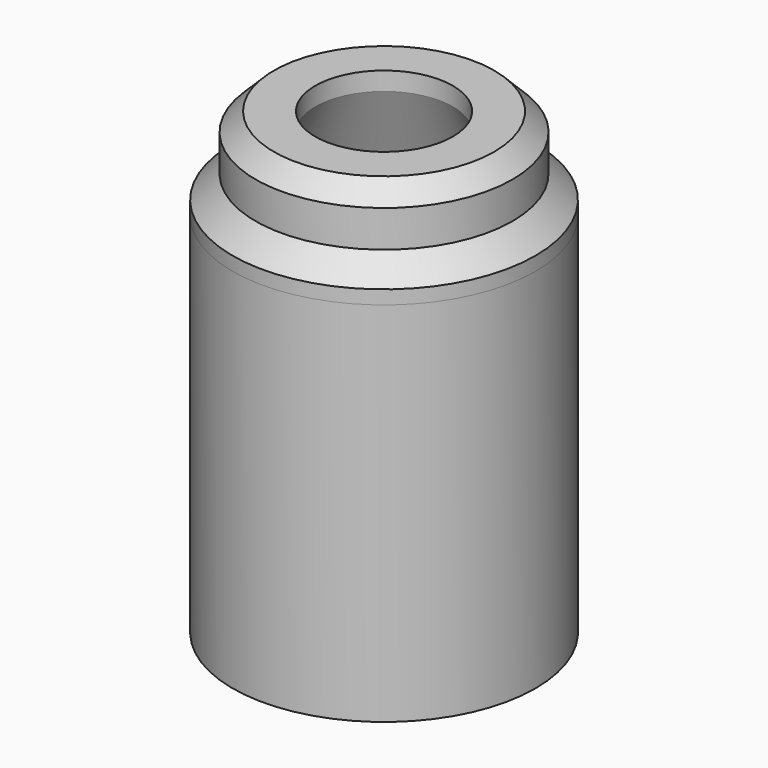
from build123d import *

# Parameters (mm, degrees)
F0_R          = 16.5
F0_R_2        = 14
F1_DEPTH      = 40
F2_R          = 14
F2_R_2        = 7.5
F3_DEPTH      = 10
F3_DEPTH_BACK = 5
F4_S5_R       = 16.5
F4_T6_DEPTH   = 27
F5_SIZE       = 2
F6_S5_R       = 14
F6_T6_DEPTH   = 24
F7_SIZE       = 5


# Not quite as in the source:
# - a fillet or chamfer that OpenCascade refuses, or shapes differently, is made with other operations: its cross-section is extruded or revolved along the edge and cut away or added


with BuildPart() as f1:
    # F0 (on Top) → F1 (new body)
    with BuildSketch(Plane.XY):
        Circle(F0_R)
        Circle(F0_R_2, mode=Mode.SUBTRACT)
    extrude(amount=F1_DEPTH)

    # F2 (on face) → F3 (join, two sides)
    with BuildSketch(Plane.XY.offset(40)) as f3_sk:
        Circle(F2_R)
        Circle(F2_R_2, mode=Mode.SUBTRACT)
    extrude(amount=F3_DEPTH)
    extrude(f3_sk.sketch, amount=-F3_DEPTH_BACK)

    # F4: chamfer of 4 on 1 edges, made by hand


with BuildPart() as f4_tool2:
    # F4_s3 → F4_t4 (revolve)
    with BuildSketch(Plane.XZ):
        Polygon((18, 40), (14, 44), (14, 40), align=None)
    revolve(axis=Axis((0, 0, 40), (0, 0, 1)))

    # F4_s5 → F4_t6 (intersect, symmetric)
    with BuildSketch(Plane.XY.offset(42)):
        Circle(F4_S5_R)
    extrude(amount=F4_T6_DEPTH, both=True, mode=Mode.INTERSECT)


with BuildPart() as f1_1:
    add(f1.part)

    # F4_t1: union F4_tool2
    add(f4_tool2.part)

    # F5
    f5_edges = [f1_1.edges().sort_by_distance(p)[0] for p in [
        (-14, 0, 50),
    ]]
    chamfer(f5_edges, length=F5_SIZE)

    # F6: chamfer of 8 on 1 edges, made by hand


with BuildPart() as f6_tool2:
    # F6_s3 → F6_t4 (revolve)
    with BuildSketch(Plane.XZ):
        Polygon((7.5, 43), (15.5, 35), (7.5, 35), align=None)
    revolve(axis=Axis((0, 0, 35), (0, 0, 1)))

    # F6_s5 → F6_t6 (intersect, symmetric)
    with BuildSketch(Plane.XY.offset(39)):
        Circle(F6_S5_R)
    extrude(amount=F6_T6_DEPTH, both=True, mode=Mode.INTERSECT)


with BuildPart() as f1_2:
    add(f1_1.part)

    # F6_t1: cut F6_tool2
    add(f6_tool2.part, mode=Mode.SUBTRACT)

    # F7
    f7_edges = [f1_2.edges().sort_by_distance(p)[0] for p in [
        (-7.5, 0, 43),
    ]]
    chamfer(f7_edges, length=F7_SIZE)


solid = f1_2.part
